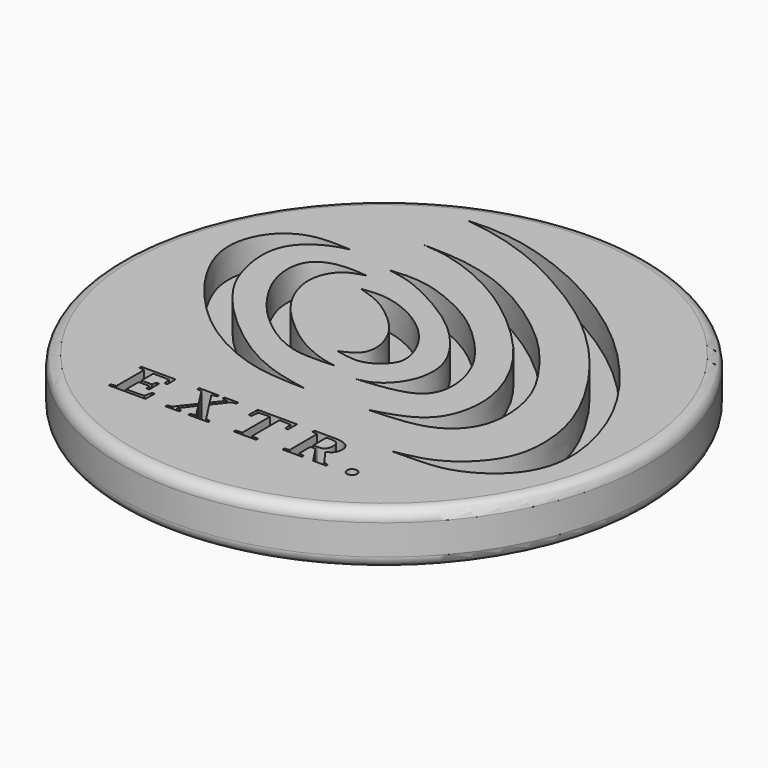
from build123d import *

# Parameters (mm, degrees)
F1_R         = 11.625
F2_DEPTH     = 2.33
F3_R         = 0.5
F5_DEPTH     = 1.3
F6_TEXT_SIZE = 2.7180417744
F7_DEPTH     = 1.3


# Not quite as in the source:
# - Text() gives the source's letters only with a copy of the font that has no kerning and outlines rounded to 1/6400 em; it was checked with that copy


with BuildPart() as f2:
    # F1 (on Top) → F2 (new body)
    with BuildSketch(Plane.XY):
        Circle(F1_R)
    extrude(amount=F2_DEPTH)

    # F3
    f3_edges = [f2.edges().sort_by_distance(p)[0] for p in [
        (-11.625, 0, 0),
        (-11.625, 0, 2.33),
    ]]
    fillet(f3_edges, radius=F3_R)

    # F4 (on face) → F5 (cut)
    with BuildSketch(Plane.XY.offset(2.33)):
        with BuildLine():
            add(Edge.make_bspline(
                [(-3.6514243693, 3.2877473859), (-3.3276815226, 3.3325111378), (-2.5933018005, 3.4340534328), (-0.9914705584, 2.8745588133), (0.4450709973, 1.603752504), (0.9273149036, 0.1665294085), (0.6374190829, -0.4442177434), (-0.1744360831, -1.0818636747), (-0.9194873385, -0.9302965694), (-1.3112876914, -0.850591925)],
                knots=[0, 0, 0, 0, 0.1318535413, 0.2990971631, 0.4812929975, 0.6345437478, 0.7360580566, 0.8612007619, 1, 1, 1, 1], degree=3))
            add(Edge.make_bspline(
                [(-3.6514243693, 3.2877473859), (-3.3018709278, 3.1827767642), (-2.5726130596, 2.9552364615), (-1.5682205984, 2.1716284826), (-0.8369721404, 1.4330660349), (-0.3843706887, 0.24822012), (-0.6522141597, -0.5081605095), (-1.0785099056, -0.6956577285), (-1.2874744643, -0.7875762531)],
                knots=[0, 0, 0, 0, 0.177810722, 0.3651808935, 0.5384733428, 0.7226715966, 0.8637256848, 1, 1, 1, 1], degree=3))
            add(Edge.make_bspline(
                [(-1.2874744643, -0.7875762531), (-1.3194903731, -0.7990705781), (-1.4202028979, -0.8354101446), (-1.3112876914, -0.850591925)],
                knots=[0, 0, 0, 0, 0.0673650109, 0.0673650109, 0.0673650109, 0.0673650109], degree=3))
        make_face()
        with BuildLine():
            add(Edge.make_bspline(
                [(-4.1191787459, 4.182448145), (-4.4173661337, 4.0994820354), (-5.0378335691, 3.9242156719), (-5.5798658255, 2.8607212444), (-5.2805487496, 1.5789037682), (-4.6266292862, 0.56580312), (-3.8009073927, -0.2373817507), (-2.7057901409, -1.1181528135), (-1.4125920225, -1.6598487408), (-0.9284782233, -1.7177741573), (-0.7310274523, -1.7413997557)],
                knots=[0, 0, 0, 0, 0.1127325401, 0.2346378394, 0.368062905, 0.4971775344, 0.623343693, 0.7650440839, 0.9041600154, 1, 1, 1, 1], degree=3))
            add(Edge.make_bspline(
                [(-4.1191787459, 4.182448145), (-4.5192853454, 4.2186256125), (-5.2994439853, 4.2891943834), (-6.4605746358, 3.8629970002), (-6.6694123921, 2.3814127895), (-5.8018935, 0.6621968646), (-4.4937925827, -0.7567525504), (-2.6726045681, -1.9001913907), (-1.3603863394, -1.765262377), (-0.7310274523, -1.7413997557)],
                knots=[0, 0, 0, 0, 0.1236832037, 0.2406555558, 0.3687863419, 0.5242181692, 0.6826764248, 0.8443692899, 1, 1, 1, 1], degree=3))
        make_face()
        with BuildLine():
            add(Edge.make_bspline(
                [(-5.7392327581, 5.3460285999), (-6.0058469599, 5.2984570506), (-6.5481631427, 5.1410858577), (-7.4712424514, 4.5644589136), (-8.0152847973, 3.4577578102), (-7.7038481231, 1.6292165288), (-7.0057036253, 0.3351459484), (-5.7699473066, -1.0922160809), (-3.7349194878, -2.7089766894), (-1.9946707331, -3.4339137423), (-0.9995238011, -3.6239304117), (-0.5455923965, -3.7055206485)],
                knots=[0, 0, 0, 0, 0.081847815, 0.1735354806, 0.2705877119, 0.3907123662, 0.4996741022, 0.6229057222, 0.7685652426, 0.8922575866, 1, 1, 1, 1], degree=3))
            add(Edge.make_bspline(
                [(-5.7392327581, 5.3460285999), (-6.362434154, 5.383883121), (-7.5617951917, 5.4567347513), (-8.9170666256, 4.4492223074), (-9.3782892142, 2.7465952818), (-8.6873878316, 1.0474755415), (-7.6048653526, -0.4893676609), (-5.793233126, -2.3058636311), (-3.0555750632, -3.659146897), (-1.3550049854, -3.6905661635), (-0.5455923965, -3.7055206485)],
                knots=[0, 0, 0, 0, 0.1169765592, 0.2251232561, 0.3365641599, 0.4522261047, 0.5716603583, 0.7113413007, 0.8626084346, 1, 1, 1, 1], degree=3))
        make_face()
        with BuildLine():
            add(Edge.make_bspline(
                [(-3.7326766178, 4.9879415892), (-3.2947413373, 5.0266090961), (-2.3664925371, 5.1085695137), (-0.7436524384, 4.5517310818), (0.7427387447, 3.7547645302), (2.2299514939, 2.3186636226), (3.0976422931, 1.0422933364), (3.4643058824, -0.4856269987), (2.9586239368, -1.8319711303), (1.3162606548, -1.9837581385), (0.3669769503, -2.0712323021)],
                knots=[0, 0, 0, 0, 0.1124397911, 0.2375457684, 0.3646081647, 0.5028110786, 0.623954148, 0.7423543473, 0.846596698, 1, 1, 1, 1], degree=3))
            add(Edge.make_bspline(
                [(-3.7326766178, 4.9879415892), (-3.3957113888, 4.9294676955), (-2.6662040965, 4.7978896565), (-1.3819411724, 4.1666944539), (-0.2268934353, 3.4786718006), (1.0255064727, 2.4602203609), (2.2895490982, 0.7106080071), (2.0678180094, -1.0009407926), (1.1402104835, -1.9443243036), (0.6026368334, -2.0325540877), (0.3669769503, -2.0712323021)],
                knots=[0, 0, 0, 0, 0.1108094458, 0.2382438411, 0.3624287484, 0.4990704141, 0.6537705832, 0.7893824223, 0.9076085, 1, 1, 1, 1], degree=3))
        make_face()
        with BuildLine():
            add(Edge.make_bspline(
                [(-4.0123036597, 7.1960231289), (-3.4437048491, 7.185015849), (-2.2727839171, 7.1623484528), (-0.3585944717, 6.6972400307), (1.6787162041, 5.5902829253), (3.7300258648, 3.9601488112), (5.0880305418, 2.2080043287), (6.0893677728, 0.5109155859), (6.3018075547, -1.9697090233), (4.8041416905, -3.4986195212), (3.0969763889, -3.5565679008), (2.1707136184, -3.58800916)],
                knots=[0, 0, 0, 0, 0.0992779335, 0.2044439916, 0.3198269282, 0.4424836297, 0.5544912585, 0.6607142818, 0.7752941118, 0.8780805243, 1, 1, 1, 1], degree=3))
            add(Edge.make_bspline(
                [(-4.0123036597, 7.1960231289), (-3.6567635838, 7.1747114787), (-2.8320115928, 7.1132738902), (-0.9447947131, 6.438781899), (1.0979148415, 5.2059854053), (3.4503955592, 3.0439618921), (4.6079609344, 1.0124433976), (5.0398032072, -0.8366047017), (4.4741864467, -2.9290044897), (2.9504060424, -3.3921117364), (2.1707136184, -3.58800916)],
                knots=[0, 0, 0, 0, 0.0923622467, 0.2126774959, 0.3480116623, 0.5022058393, 0.633712613, 0.7510506254, 0.8699017757, 0.9999404828, 0.9999404828, 0.9999404828, 0.9999404828], degree=3))
        make_face()
        with BuildLine():
            add(Edge.make_bspline(
                [(-3.9911643541, 9.5502620824), (-3.2934092397, 9.6001933548), (-1.8351301651, 9.5790898063), (0.3834021379, 8.8896162192), (2.4002487459, 7.9822804505), (5.5027122207, 5.9779710222), (8.3316142911, 2.771140383), (9.6330957076, -0.0952583084), (9.9649702579, -2.692474946), (8.9573610333, -4.4258758876), (7.1469876859, -5.4581679161), (6.1828515169, -5.4811743209), (4.7304003221, -5.4974863664)],
                knots=[0.0064868072, 0.0064868072, 0.0064868072, 0.0064868072, 0.0926346181, 0.1863113439, 0.277674262, 0.3957496264, 0.5238144687, 0.6332651491, 0.730085814, 0.8146033076, 0.8965064136, 0.9951951002, 0.9951951002, 0.9951951002, 0.9951951002], degree=3))
            add(Edge.make_bspline(
                [(-3.9911643541, 9.5502620824), (-3.5397098193, 9.4953180433), (-2.4692125128, 9.3525778475), (-0.3653601147, 8.6695935965), (1.823047392, 7.466268902), (3.9061178735, 6.0876987524), (6.2323438341, 3.7543199305), (7.9441735308, 0.9062259983), (8.4912703663, -1.1354547019), (8.409349061, -3.3963498477), (6.622852404, -5.169442424), (5.3180234165, -5.3859877457), (4.7304003221, -5.4974863664)],
                knots=[0.0094268489, 0.0094268489, 0.0094268489, 0.0094268489, 0.0820580798, 0.1797305686, 0.2820633967, 0.3841893393, 0.5022282152, 0.6199514319, 0.713495273, 0.8077497975, 0.9077735634, 0.9900726583, 0.9900726583, 0.9900726583, 0.9900726583], degree=3))
        make_face()
    extrude(amount=-F5_DEPTH, mode=Mode.SUBTRACT)

    # F6 (on face) → F7 (cut)
    with BuildSketch(Plane.XY.offset(2.33)):
        with Locations((-5.9728454801, -7.7419510691)):
            Text('E X T R .', F6_TEXT_SIZE, font='Tinos', font_style=FontStyle.BOLD, text_align=(TextAlign.LEFT, TextAlign.BOTTOM))
    extrude(amount=-F7_DEPTH, mode=Mode.SUBTRACT)


solid = f2.part
